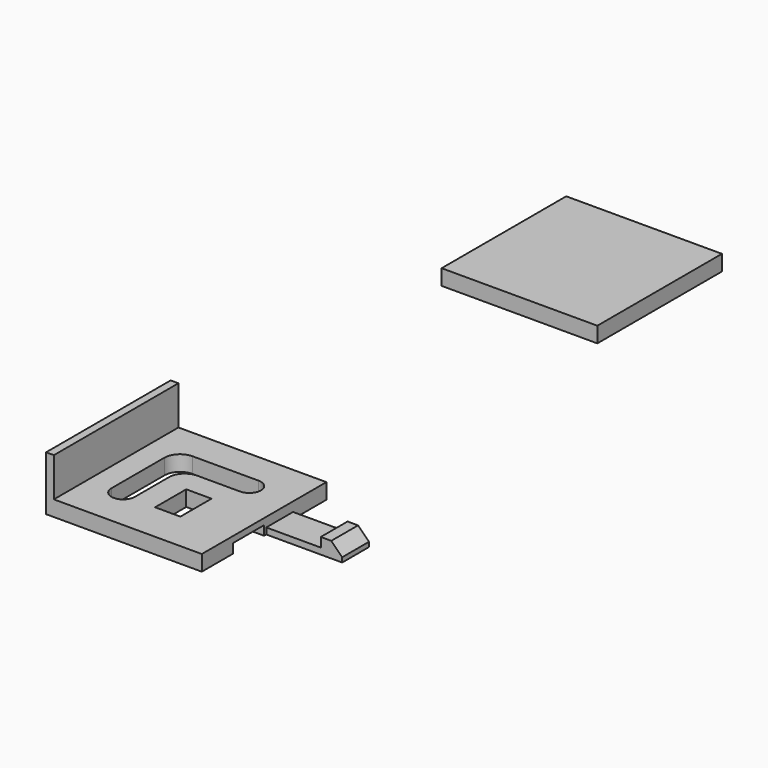
from build123d import *

# Parameters (mm, degrees)
F0_W      = 20
F0_H      = 20
F1_DEPTH  = 2
F2_W      = 5
F2_H      = 1.2
F3_DEPTH  = 10
F4_W      = 3.25
F4_H      = 5
F5_DEPTH  = 0.801
F6_W      = 4.3
F6_H      = 0.8
F7_DEPTH  = 9.75
F8_W      = 2.75
F8_H      = 4.3
F9_DEPTH  = 1.2
F10_SIZE  = 1.4
F11_W     = 1
F11_H     = 20
F12_DEPTH = 5
F14_DEPTH = 2.001
F15_R     = 2
F16_R     = 1.49999


# Not quite as in the source:
# - a fillet or chamfer is up to 0.001 mm smaller than in the source, because OpenCascade refuses the exact size


with BuildPart() as f1:
    # F0 (on Top) → F1 (new body)
    with BuildSketch(Plane.XY):
        with Locations((10.8443908393, -31.3820495651)):
            Rectangle(F0_W, F0_H)
    extrude(amount=F1_DEPTH)

    # F2 (on face) → F3 (cut)
    with BuildSketch(Plane.YZ.offset(20.8443908393)):
        with Locations((-33.8820495651, 0.6)):
            Rectangle(F2_W, F2_H)
    extrude(amount=-F3_DEPTH, mode=Mode.SUBTRACT)

    # F4 (on face) → F5 (cut, through all)
    with BuildSketch(Plane(origin=(0, 0, 1.2), x_dir=(1, 0, 0), z_dir=(0, 0, -1))):
        with Locations((12.4693908393, 33.8820495651)):
            Rectangle(F4_W, F4_H)
    extrude(amount=-F5_DEPTH, mode=Mode.SUBTRACT)

    # F6 (on face) → F7 (join)
    with BuildSketch(Plane.YZ.offset(20.8443908393)):
        with Locations((-28.8820495651, 0.4)):
            Rectangle(F6_W, F6_H)
    extrude(amount=F7_DEPTH)

    # F8 (on face) → F9 (join)
    with BuildSketch(Plane.XY.offset(0.8)):
        with Locations((29.2193908393, -28.8820495651)):
            Rectangle(F8_W, F8_H)
    extrude(amount=F9_DEPTH)

    # F10
    f10_edges = [f1.edges().sort_by_distance(p)[0] for p in [
        (30.594391, -28.88205, 2),
    ]]
    chamfer(f10_edges, length=F10_SIZE)

    # F11 (on face) → F12 (join)
    with BuildSketch(Plane.XY.offset(2)):
        with Locations((1.3443908393, -31.3820495651)):
            Rectangle(F11_W, F11_H)
    extrude(amount=F12_DEPTH)

    # F13 (on face) → F14 (cut, through all)
    with BuildSketch(Plane.XY.offset(2)):
        Polygon((4.8443908393, -25.3820495651), (4.8443908393, -37.3820495651), (7.8443908393, -37.3820495651), (7.8443908393, -28.3820495651), (16.8443908393, -28.3820495651), (16.8443908393, -25.3820495651), align=None)
    extrude(amount=-F14_DEPTH, mode=Mode.SUBTRACT)

    # F15
    f15_edges = [f1.edges().sort_by_distance(p)[0] for p in [
        (7.844391, -28.38205, 1),
        (4.844391, -25.38205, 1),
    ]]
    fillet(f15_edges, radius=F15_R)

    # F16 (radius 1.5 in the source; OpenCascade refuses exactly that, so slightly less here)
    f16_edges = [f1.edges().sort_by_distance(p)[0] for p in [
        (4.844391, -37.38205, 1),
        (7.844391, -37.38205, 1),
        (16.844391, -28.38205, 1),
        (16.844391, -25.38205, 1),
    ]]
    fillet(f16_edges, radius=F16_R)


with BuildPart() as f1b:
    # F0 (on Top) → F1, piece 2 (new body)
    with BuildSketch(Plane.XY):
        with Locations((10.8443908393, 32.1213992728)):
            Rectangle(F0_W, F0_H)
    extrude(amount=F1_DEPTH)


solid = Compound([f1.part, f1b.part])
